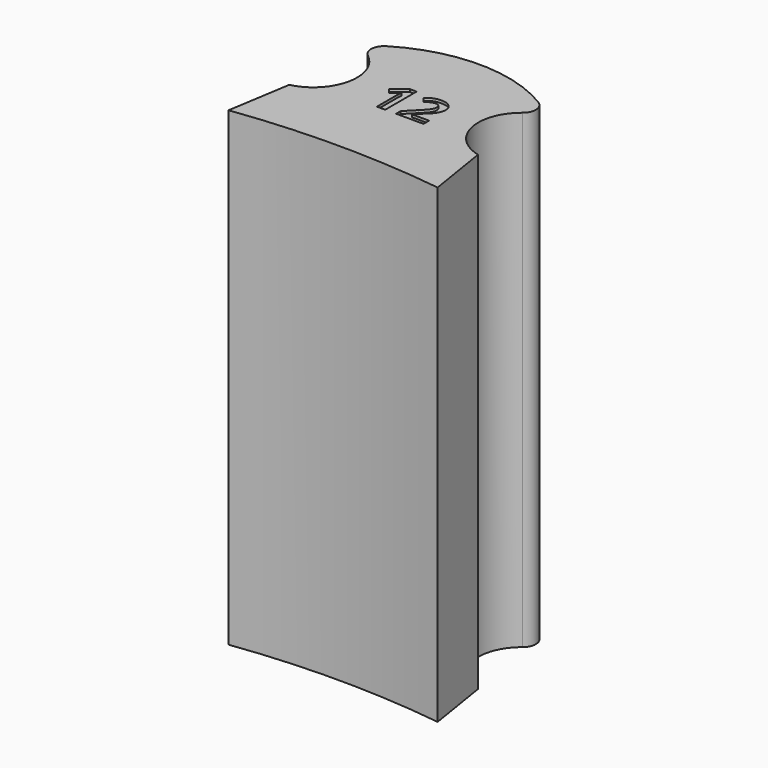
from build123d import *

# Parameters (mm, degrees)
F1_DEPTH     = 180
F2_TEXT_SIZE = 21.0426799539
F3_DEPTH     = 1


# Not quite as in the source:
# - Text() gives the source's letters only with a copy of the font that has no kerning and outlines rounded to 1/6400 em; it was checked with that copy


with BuildPart() as f1:
    # F0 (on Top) → F1 (new body)
    with BuildSketch(Plane.XY):
        with BuildLine():
            Line((3.8687128108, 24.1569802165), (0, 0))
            ThreePointArc((0, 0), (40, 2.6430687706), (80, 0))
            Line((80, 0), (76.1312871892, 24.1569802165))
            ThreePointArc((76.1312871892, 24.1569802165), (63.5975554576, 36.8458138953), (69.5972800683, 53.6417728094))
            ThreePointArc((69.5972800683, 53.6417728094), (71.4969098635, 57.8715436357), (69.1043731597, 61.843359684))
            ThreePointArc((69.1043731597, 61.843359684), (40, 70), (10.8956268403, 61.843359684))
            ThreePointArc((10.8956268403, 61.843359684), (8.5030901365, 57.8715436357), (10.4027199317, 53.6417728094))
            ThreePointArc((10.4027199317, 53.6417728094), (16.4024445424, 36.8458138953), (3.8687128108, 24.1569802165))
        make_face()
    extrude(amount=F1_DEPTH)

    # F2 (on face) → F3 (cut)
    with BuildSketch(Plane.XY.offset(180)):
        with Locations((27.6407134458, 29.5085348189)):
            Text('12', F2_TEXT_SIZE, font='Open Sans', font_style=FontStyle.BOLD, text_align=(TextAlign.LEFT, TextAlign.BOTTOM))
    extrude(amount=-F3_DEPTH, mode=Mode.SUBTRACT)


solid = f1.part
